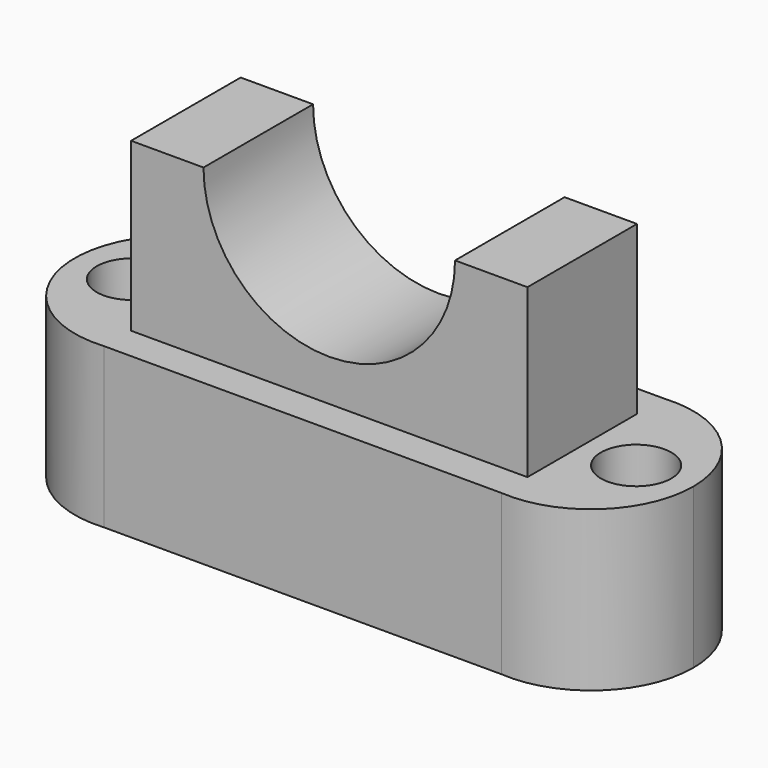
from build123d import *

# Parameters (mm, degrees)
F1_DEPTH = 31.75
F2_R     = 7.0115347254
F3_DEPTH = 31.751
F4_W     = 78.8504332304
F4_H     = 27.2497832775
F5_DEPTH = 33.274
F7_DEPTH = 33.9844357044


# Not quite as in the source:
# - a feature of the source that left no trace in its solid (it failed there, or was rolled back) is left out


with BuildPart() as f1:
    # F0 (on Top) → F1 (new body)
    with BuildSketch(Plane.XY):
        with BuildLine():
            Line((39.576777419, 20.2923920006), (-39.5247050543, 20.2923920006))
            ThreePointArc((-39.5247050543, 20.2923920006), (-26.2003502762, 13.8037157784), (-20.8060217658, 0))
            ThreePointArc((-20.8060217658, 0), (-26.2003502762, -13.8037157784), (-39.5247050543, -20.2923920006))
            Line((-39.5247050543, -20.2923920006), (39.576777419, -20.2923920006))
            ThreePointArc((39.576777419, -20.2923920006), (20.8101499679, 0), (39.576777419, 20.2923920006))
        make_face()
        with BuildLine():
            Line((-39.5247050543, 20.2923920006), (-41.1645658314, 20.2923920006))
            Line((-41.1645658314, 20.2923920006), (-41.1645658314, -20.2923920006))
            Line((-41.1645658314, -20.2923920006), (-39.5247050543, -20.2923920006))
            ThreePointArc((-39.5247050543, -20.2923920006), (-26.2003502762, -13.8037157784), (-20.8060217658, 0))
            ThreePointArc((-20.8060217658, 0), (-26.2003502762, 13.8037157784), (-39.5247050543, 20.2923920006))
        make_face()
        with BuildLine():
            Line((-41.1645658314, -20.2923920006), (-41.1645658314, 20.2923920006))
            Line((-41.1645658314, 20.2923920006), (-39.5247050543, 20.2923920006))
            ThreePointArc((-39.5247050543, 20.2923920006), (-61.5231098971, 0), (-39.5247050543, -20.2923920006))
            Line((-39.5247050543, -20.2923920006), (-41.1645658314, -20.2923920006))
        make_face()
        with BuildLine():
            Line((41.1645658314, 20.2923920006), (39.576777419, 20.2923920006))
            ThreePointArc((39.576777419, 20.2923920006), (20.8101499679, 0), (39.576777419, -20.2923920006))
            Line((39.576777419, -20.2923920006), (41.1645658314, -20.2923920006))
            Line((41.1645658314, -20.2923920006), (41.1645658314, 20.2923920006))
        make_face()
        with BuildLine():
            ThreePointArc((61.518981695, 0), (54.9845466472, 14.9435730466), (39.576777419, 20.2923920006))
            Line((39.576777419, 20.2923920006), (41.1645658314, 20.2923920006))
            Line((41.1645658314, 20.2923920006), (41.1645658314, -20.2923920006))
            Line((41.1645658314, -20.2923920006), (39.576777419, -20.2923920006))
            ThreePointArc((39.576777419, -20.2923920006), (54.9845466472, -14.9435730466), (61.518981695, 0))
        make_face()
    extrude(amount=F1_DEPTH)

    # F2 (on face) → F3 (cut, through all)
    with BuildSketch(Plane.XY.offset(31.75)):
        with Locations((50.1511953771, 0)):
            Circle(F2_R)
        with Locations((-50.1511953771, 0)):
            Circle(F2_R)
    extrude(amount=-F3_DEPTH, mode=Mode.SUBTRACT)

    # F4 (on face) → F5 (join)
    with BuildSketch(Plane.XY.offset(31.75)):
        Rectangle(F4_W, F4_H)
    extrude(amount=F5_DEPTH)

    # F6 (on face) → F7 (cut, through all)
    with BuildSketch(Plane.XZ.offset(13.6248916388)):
        with BuildLine():
            ThreePointArc((-25.020677247, 65.024), (0, 40.003322753), (25.020677247, 65.024))
            Line((25.020677247, 65.024), (-25.020677247, 65.024))
        make_face()
    extrude(amount=-F7_DEPTH, mode=Mode.SUBTRACT)


solid = f1.part
